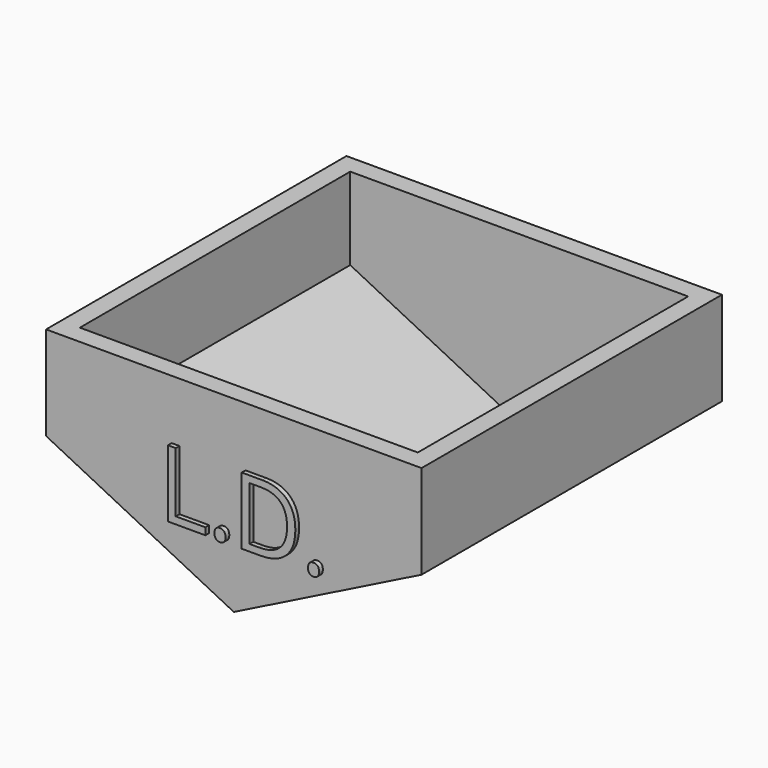
from build123d import *

# Parameters (mm, degrees)
F1_DEPTH     = 50.8
F2_T         = -2.54
F3_TEXT_SIZE = 12.7181152089
F4_DEPTH     = 0.635


# Not quite as in the source:
# - Text() gives the source's letters only with a copy of the font that has no kerning and outlines rounded to 1/6400 em; it was checked with that copy


with BuildPart() as f1:
    # F0 (on Front) → F1 (new body)
    with BuildSketch(Plane.XZ):
        Polygon((8.6414335847, 37.1010734975), (-42.1585664153, 37.1010734975), (-42.1585664153, 24.4010734975), (-16.7585664153, 11.7010734975), (8.6414335847, 24.4010734975), align=None)
    extrude(amount=F1_DEPTH)

    # F2
    f2_openings = [f1.faces().sort_by_distance(p)[0] for p in [
        (-16.758566, -25.4, 37.101073),
    ]]
    offset(amount=F2_T, openings=f2_openings)

    # F3 (on face) → F4 (join)
    with BuildSketch(Plane.XZ.offset(50.8)):
        with Locations((-26.4116935432, 20.0047045946)):
            Text('L.D.', F3_TEXT_SIZE, font='Open Sans', text_align=(TextAlign.LEFT, TextAlign.BOTTOM))
    extrude(amount=F4_DEPTH)


solid = f1.part
